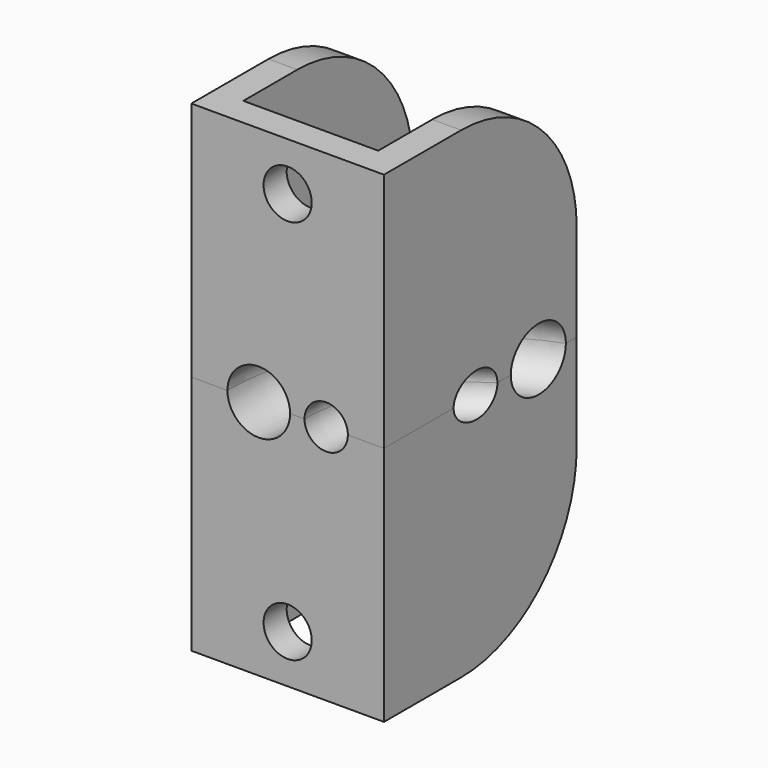
from build123d import *

# Parameters (mm, degrees)
F2_W           = 20
F2_H           = 50
F3_DEPTH       = 25
F5_START       = -3
F4_W           = 14
F4_H           = 21
F5_DEPTH       = 22.001
F1_R           = 3.25
F6_ANGLE       = 90
F1_R_2         = 2.25
F7_ANGLE       = 90
F8_R           = 2.5
F9_DEPTH       = 25
F10_R          = 1.9619906376
F11_DEPTH      = 25
F11_DEPTH_BACK = 25
F12_W          = 35.8874800149
F12_H          = 25.5419854075
F13_DEPTH      = 25
F14_R          = 15


with BuildPart() as f3:
    # F2 (on Front) → F3 (new body)
    with BuildSketch(Plane.XZ):
        with Locations((-19, 0)):
            Rectangle(F2_W, F2_H)
    extrude(amount=-F3_DEPTH)

    # F4 (on Front) → F5 (cut)
    with BuildSketch(Plane.XZ.offset(F5_START)):
        with Locations((-19, 15.5)):
            Rectangle(F4_W, F4_H)
    extrude(amount=-F5_DEPTH, mode=Mode.SUBTRACT)

    # F1 (on Right) → F6 (revolve, cut)
    with BuildSketch(Plane.YZ):
        with Locations((22, 0)):
            Circle(F1_R)
    revolve(axis=Axis((0, 0, 0), (0, 0, 1)), revolution_arc=F6_ANGLE, mode=Mode.SUBTRACT)

    # F1 (on Right) → F7 (revolve, cut)
    with BuildSketch(Plane.YZ):
        with Locations((15, 0)):
            Circle(F1_R_2)
    revolve(axis=Axis((0, 0, 0), (0, 0, 1)), revolution_arc=F7_ANGLE, mode=Mode.SUBTRACT)

    # F8 (on Front) → F9 (cut)
    with BuildSketch(Plane.XZ):
        with Locations((-19, 20)):
            Circle(F8_R)
    extrude(amount=-F9_DEPTH, mode=Mode.SUBTRACT)

    # F10 (on Top) → F11 (cut, two sides)
    with BuildSketch(Plane.XY) as f11_sk:
        with Locations((-19, 21)):
            Circle(F10_R)
    extrude(amount=-F11_DEPTH, mode=Mode.SUBTRACT)
    extrude(f11_sk.sketch, amount=F11_DEPTH_BACK, mode=Mode.SUBTRACT)

    # F12 (on Front) → F13 (cut)
    with BuildSketch(Plane.XZ):
        with Locations((-20.9509915439, -12.7709927037)):
            Rectangle(F12_W, F12_H)
    extrude(amount=-F13_DEPTH, mode=Mode.SUBTRACT)

    # F14
    f14_edges = [f3.edges().sort_by_distance(p)[0] for p in [
        (-10.5, 25, 25),
        (-27.5, 25, 25),
    ]]
    fillet(f14_edges, radius=F14_R)


with BuildPart() as f15_1:
    # F15: instance of F3
    add(f3.part.mirror(Plane.XY))


solid = Compound([f3.part, f15_1.part])
